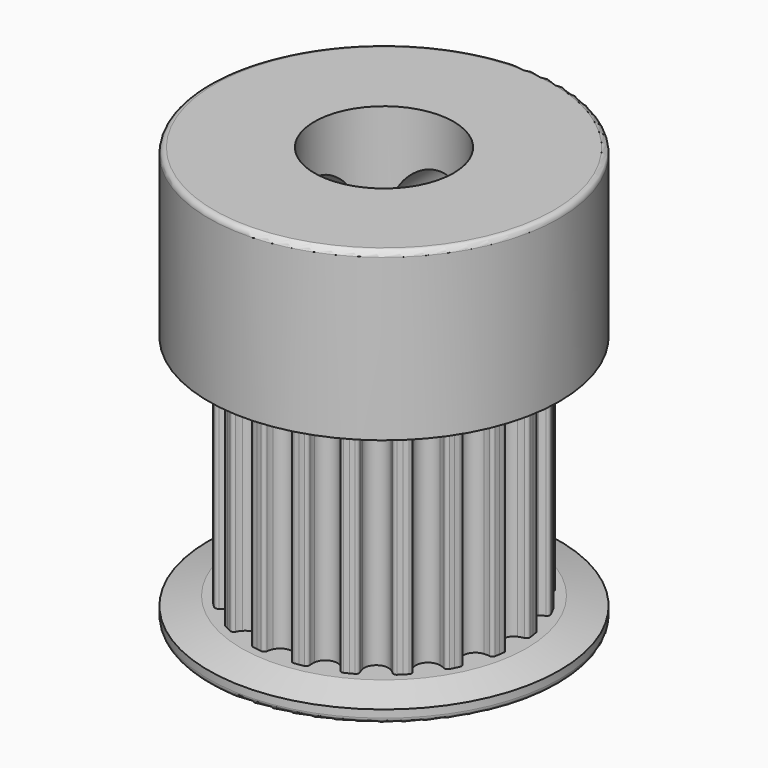
from build123d import *

# Parameters (mm, degrees)
F3_DEPTH    = 5
F4_COUNT    = 20
F5_R        = 8
F6_DEPTH    = 1
F7_R        = 8
F8_DEPTH    = 1
F9_R        = 8
F10_DEPTH   = 7
F11_R       = 3.175
F12_DEPTH   = 19.001
F13_R       = 1.75
F14_DEPTH   = 8.001
F15_R       = 1.75
F16_DEPTH   = 8.0010001
F17_SIZE2   = 0.4019237886
F17_SIZE    = 1.5
F17_2_SIZE2 = 0.4019237886
F17_2_SIZE  = 1.5
F18_R       = 0.25


# Not quite as in the source:
# - a feature names something its author has since deleted; it is built from what else it names


with BuildPart() as f3:
    # F2 (on Top) → F3 (new body, symmetric)
    with BuildSketch(Plane.XY):
        with BuildLine():
            ThreePointArc((0.5072317048, 5.6927824446), (0.3024954694, 5.4527213714), (0, 5.3630400697))
            ThreePointArc((0, 5.3630400697), (-0.3024954694, 5.4527213714), (-0.5072317048, 5.6927824446))
            ThreePointArc((-0.5072317048, 5.6927824446), (-0.5520948337, 5.8145502635), (-0.5808117717, 5.9411023854))
            ThreePointArc((-0.5808117717, 5.9411023854), (-0.6387574174, 6.037333963), (-0.7472774352, 6.0663446529))
            ThreePointArc((-0.7472774352, 6.0663446529), (-0.8518447388, 6.0525466999), (-0.9561583811, 6.0369464271))
            Line((-0.9561583811, 6.0369464271), (0, 0))
            Line((0, 0), (0.9561583811, 6.0369464271))
            ThreePointArc((0.9561583811, 6.0369464271), (0.8518447388, 6.0525466999), (0.7472774352, 6.0663446529))
            ThreePointArc((0.7472774352, 6.0663446529), (0.6387574174, 6.037333963), (0.5808117717, 5.9411023854))
            ThreePointArc((0.5808117717, 5.9411023854), (0.5520948337, 5.8145502635), (0.5072317048, 5.6927824446))
        make_face()
    extrude(amount=F3_DEPTH, both=True)

    # F4: F3 ×20 about axis
    f4_axis = Axis((0, 0, 0), (0, 0, -1))


with BuildPart() as f3_1:
    add(f3.part)
    for i in range(1, F4_COUNT):
        add(f3.part.rotate(f4_axis, i * 360 / F4_COUNT))

    # F5 (on face) → F6 (join)
    with BuildSketch(Plane(origin=(0, 0, -5), x_dir=(1, 0, 0), z_dir=(0, 0, -1))):
        Circle(F5_R)
    extrude(amount=F6_DEPTH)

    # F7 (on face) → F8 (join)
    with BuildSketch(Plane.XY.offset(5)):
        Circle(F7_R)
    extrude(amount=F8_DEPTH)

    # F9 (on face) → F10 (join)
    with BuildSketch(Plane.XY.offset(6)):
        Circle(F9_R)
    extrude(amount=F10_DEPTH)

    # F11 (on face) → F12 (cut, through all)
    with BuildSketch(Plane.XY.offset(13)):
        Circle(F11_R)
    extrude(amount=-F12_DEPTH, mode=Mode.SUBTRACT)

    # F13 (on Front) → F14 (cut, through all)
    with BuildSketch(Plane.XZ):
        with Locations((0, 9)):
            Circle(F13_R)
    extrude(amount=-F14_DEPTH, mode=Mode.SUBTRACT)

    # F15 (on Right) → F16 (cut, through all)
    with BuildSketch(Plane.YZ):
        with Locations((0, 9)):
            Circle(F15_R)
    extrude(amount=-F16_DEPTH, mode=Mode.SUBTRACT)

    # F17
    f17_edges = [f3_1.edges().sort_by_distance(p)[0] for p in [
        (-8, 0, -5),
    ]]
    f17_side = f3_1.faces().sort_by_distance((-7.773726, 0, -5))[0]
    chamfer(f17_edges, length=F17_SIZE, length2=F17_SIZE2, reference=f17_side)

    # F17#2
    f17_2_edges = [f3_1.edges().sort_by_distance(p)[0] for p in [
        (-8, 0, 5),
    ]]
    f17_2_side = f3_1.faces().sort_by_distance((-7.773726, 0, 5))[0]
    chamfer(f17_2_edges, length=F17_2_SIZE, length2=F17_2_SIZE2, reference=f17_2_side)

    # F18
    f18_edges = [f3_1.edges().sort_by_distance(p)[0] for p in [
        (-8, 0, 13),
        (-8, 0, -6),
    ]]
    fillet(f18_edges, radius=F18_R)


solid = f3_1.part
